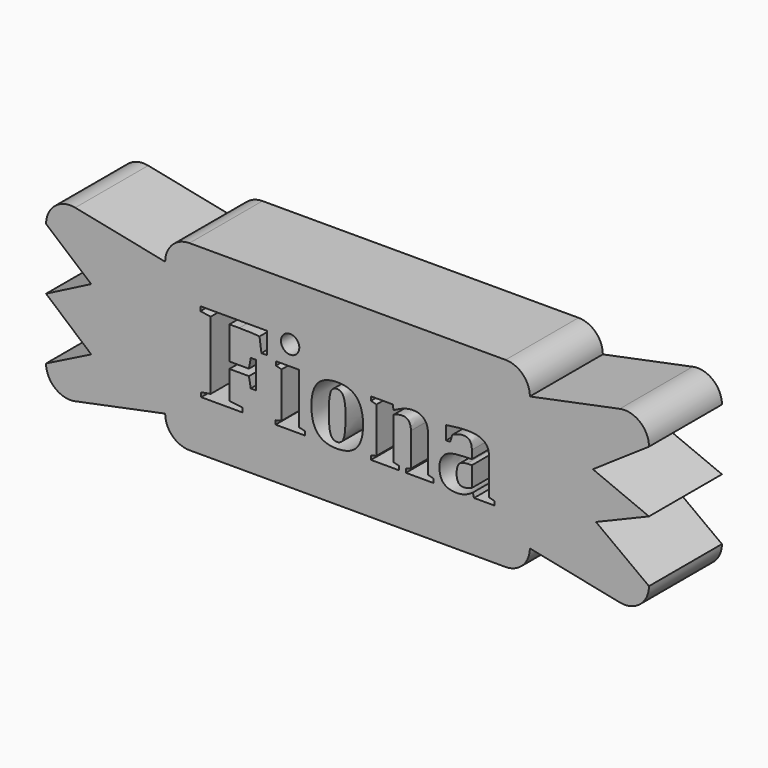
from build123d import *

# Parameters (mm, degrees)
F1_DEPTH     = 19.05
F2_TEXT_SIZE = 25.4812213932
F3_DEPTH     = 44.196


# Not quite as in the source:
# - Text() gives the source's letters only with a copy of the font that has no kerning and outlines rounded to 1/6400 em; it was checked with that copy


with BuildPart() as f1:
    # F0 (on Front) → F1 (new body)
    with BuildSketch(Plane.XZ):
        with BuildLine():
            Line((-33.4230051324, -5.8734777119), (-33.4230051324, 22.0665222881))
            Line((-33.4230051324, 22.0665222881), (-52.2138209191, 25.9021814988))
            ThreePointArc((-52.2138209191, 25.9021814988), (-56.4426950218, 24.8597694212), (-58.3098209191, 20.9248183415))
            Line((-58.3098209191, 20.9248183415), (-48.8820485771, 12.9316626117))
            Line((-48.8820485771, 12.9316626117), (-58.3098209191, 8.0965222881))
            Line((-58.3098209191, 8.0965222881), (-48.8820485771, 0))
            Line((-48.8820485771, 0), (-58.3098209191, -4.7317737652))
            ThreePointArc((-58.3098209191, -4.7317737652), (-56.4426950218, -8.6667248449), (-52.2138209191, -9.7091369225))
            Line((-52.2138209191, -9.7091369225), (-33.4230051324, -5.8734777119))
        make_face()
        with BuildLine():
            Line((37.6969948676, 27.1465222881), (-28.3430051324, 27.1465222881))
            ThreePointArc((-28.3430051324, 27.1465222881), (-31.9351075808, 25.6586247366), (-33.4230051324, 22.0665222881))
            Line((-33.4230051324, 22.0665222881), (-33.4230051324, -5.8734777119))
            ThreePointArc((-33.4230051324, -5.8734777119), (-31.9351075808, -9.4655801603), (-28.3430051324, -10.9534777119))
            Line((-28.3430051324, -10.9534777119), (37.6969948676, -10.9534777119))
            ThreePointArc((37.6969948676, -10.9534777119), (41.2890973161, -9.4655801603), (42.7769948676, -5.8734777119))
            Line((42.7769948676, -5.8734777119), (42.7769948676, 22.0665222881))
            ThreePointArc((42.7769948676, 22.0665222881), (41.2890973161, 25.6586247366), (37.6969948676, 27.1465222881))
        make_face()
        with BuildLine():
            Line((61.5678106543, 25.9021814988), (42.7769948676, 22.0665222881))
            Line((42.7769948676, 22.0665222881), (42.7769948676, -5.8734777119))
            Line((42.7769948676, -5.8734777119), (61.5678106543, -9.7091369225))
            ThreePointArc((61.5678106543, -9.7091369225), (65.796684757, -8.6667248449), (67.6638106543, -4.7317737652))
            Line((67.6638106543, -4.7317737652), (56.5894171596, 3.473978024))
            Line((56.5894171596, 3.473978024), (67.6638106543, 8.0965222881))
            Line((67.6638106543, 8.0965222881), (55.938500911, 12.9614956677))
            Line((55.938500911, 12.9614956677), (67.6638106543, 20.9248183415))
            ThreePointArc((67.6638106543, 20.9248183415), (65.796684757, 24.8597694212), (61.5678106543, 25.9021814988))
        make_face()
    extrude(amount=F1_DEPTH)

    # F2 (on face) → F3 (cut)
    with BuildSketch(Plane.XZ.offset(19.05)):
        with Locations((-26.4917906482, -0.402652412)):
            Text('Fiona', F2_TEXT_SIZE, font='Tinos', font_style=FontStyle.BOLD, text_align=(TextAlign.LEFT, TextAlign.BOTTOM))
    extrude(amount=-F3_DEPTH, mode=Mode.SUBTRACT)


solid = f1.part
